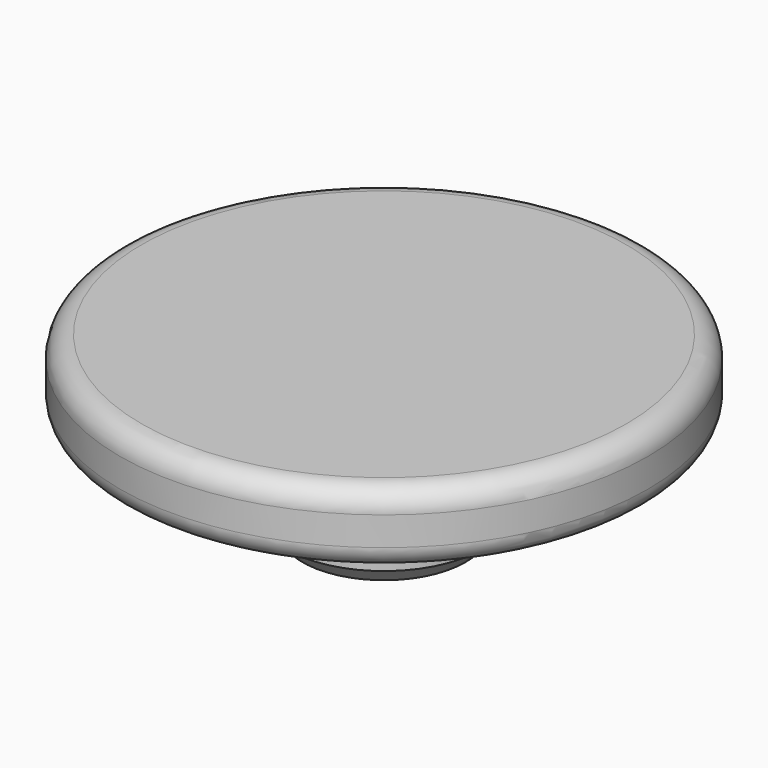
from build123d import *

# Parameters (mm, degrees)
F0_R     = 11
F0_R_2   = 5.5
F0_R_3   = 4.1
F1_DEPTH = 3
F2_DEPTH = 4.25
F3_SIZE  = 0.7
F4_R     = 0.9
F5_DEPTH = 0.5


with BuildPart() as f1:
    # F0 (on Top) → F1 (new body)
    with BuildSketch(Plane.XY):
        Circle(F0_R)
        Circle(F0_R_2, mode=Mode.SUBTRACT)
        Circle(F0_R_2)
        Circle(F0_R_3, mode=Mode.SUBTRACT)
        Circle(F0_R_3)
    extrude(amount=F1_DEPTH)

    # F0 (on Top) → F2 (join)
    with BuildSketch(Plane.XY):
        Circle(F0_R_3)
    extrude(amount=-F2_DEPTH)

    # F3
    f3_edges = [f1.edges().sort_by_distance(p)[0] for p in [
        (-4.1, 0, -4.25),
    ]]
    chamfer(f3_edges, length=F3_SIZE)

    # F4
    f4_edges = [f1.edges().sort_by_distance(p)[0] for p in [
        (11, 0, 1.5),
        (-11, 0, 0),
        (-11, 0, 3),
    ]]
    fillet(f4_edges, radius=F4_R)

    # F0 (on Top) → F5 (join)
    with BuildSketch(Plane.XY):
        Circle(F0_R_2)
        Circle(F0_R_3, mode=Mode.SUBTRACT)
    extrude(amount=-F5_DEPTH)


solid = f1.part
